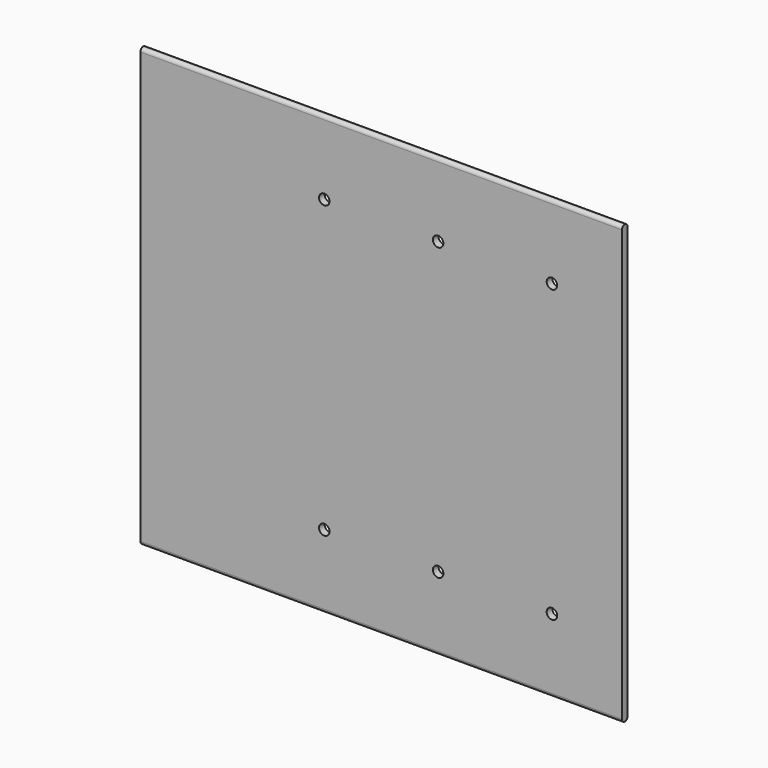
from build123d import *

# Parameters (mm, degrees)
F0_W     = 698.5
F0_H     = 635
F1_DEPTH = 10.16
F3_R     = 5.07999
F5_D     = 15.24


# Not quite as in the source:
# - a fillet or chamfer is up to 0.001 mm smaller than in the source, because OpenCascade refuses the exact size


with BuildPart() as f1:
    # F0 (on Front) → F1 (new body)
    with BuildSketch(Plane.XZ):
        with Locations((349.25, 317.5)):
            Rectangle(F0_W, F0_H)
    extrude(amount=F1_DEPTH)

    # F3 (radius 5.08 in the source; OpenCascade refuses exactly that, so slightly less here)
    f3_edges = [f1.edges().sort_by_distance(p)[0] for p in [
        (349.25, -10.16, 635),
        (349.25, 0, 635),
        (349.25, -10.16, 0),
        (349.25, 0, 0),
    ]]
    fillet(f3_edges, radius=F3_R)

    # F5 (through all)
    with Locations(Plane.XZ.offset(10.16)):
        with Locations((431.8, 528.32), (266.7, 528.32), (596.9, 528.32), (596.9, 106.68), (431.8, 106.68), (266.7, 106.68)):
            Hole(F5_D / 2)


solid = f1.part
